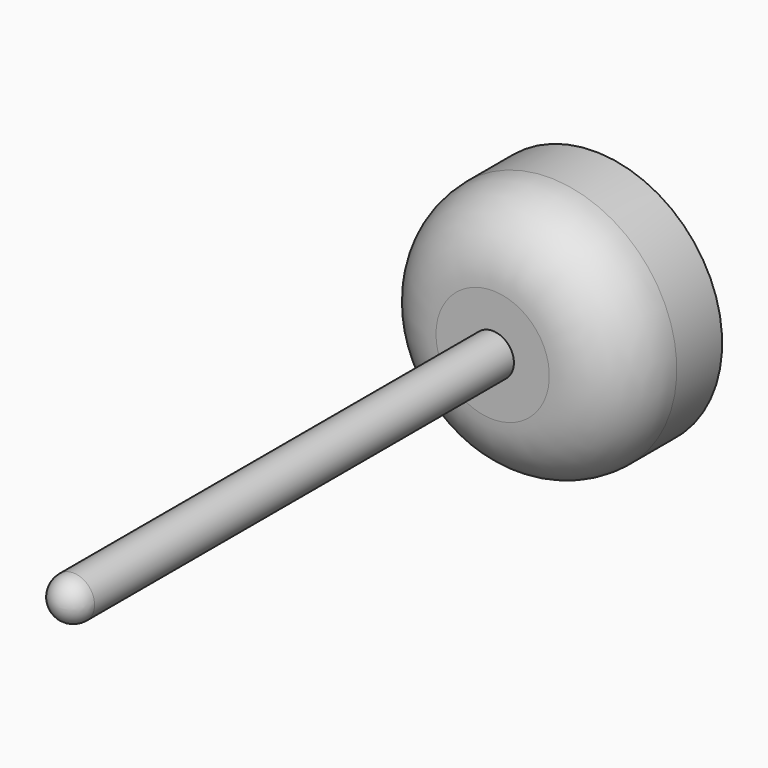
from build123d import *

# Parameters (mm, degrees)
F0_R     = 38.1
F1_DEPTH = 977.9
F2_R     = 38.1
F3_R     = 228.6
F4_DEPTH = 228.6
F5_T     = -25.4
F6_SIZE  = 50.8
F8_R     = 127
F9_SIZE  = 50.8
F10_R    = 76.2


# Not quite as in the source:
# - a fillet or chamfer that OpenCascade refuses, or shapes differently, is made with other operations: its cross-section is extruded or revolved along the edge and cut away or added


with BuildPart() as f1:
    # F0 (on Front) → F1 (new body)
    with BuildSketch(Plane.XZ):
        with Locations((-33.5694141686, 28.1756240875)):
            Circle(F0_R)
    extrude(amount=F1_DEPTH)

    # F2
    f2_edges = [f1.edges().sort_by_distance(p)[0] for p in [
        (-71.669414, -977.9, 28.175624),
    ]]
    fillet(f2_edges, radius=F2_R)


with BuildPart() as f4:
    # F3 (on face) → F4 (new body)
    with BuildSketch(Plane(origin=(0, 0, 0), x_dir=(-1, 0, 0), z_dir=(0, 1, 0))):
        with Locations((33.5694141686, 28.1756240875)):
            Circle(F3_R)
    extrude(amount=F4_DEPTH)

    # F5
    f5_openings = [f4.faces().sort_by_distance(p)[0] for p in [
        (-33.569414, 228.6, 28.175624),
    ]]
    offset(amount=F5_T, openings=f5_openings)

    # F6
    f6_edges = [f4.edges().sort_by_distance(p)[0] for p in [
        (169.630586, 25.4, 28.175624),
    ]]
    chamfer(f6_edges, length=F6_SIZE)

    # F7: chamfer of 50.8 on 3 edges, made by hand

    # F7_s1 → F7_t2 (revolve)
    with BuildSketch(Plane.XY.offset(28.1756240875)):
        Polygon((-221.8904386529, 61.3210244843), (-135.1694141686, 25.4), (-185.9694141686, 25.4), align=None)
    revolve(axis=Axis((-33.5694141686, 25.4, 28.1756240875), (0, -1, 0)))

    # F8
    f8_edges = [f4.edges().sort_by_distance(p)[0] for p in [
        (195.030586, 0, 28.175624),
    ]]
    fillet(f8_edges, radius=F8_R)

    # F9
    f9_edges = [f4.edges().sort_by_distance(p)[0] for p in [
        (68.030586, 25.4, 28.175624),
    ]]
    chamfer(f9_edges, length=F9_SIZE)

    # F10
    f10_edges = [f4.edges().sort_by_distance(p)[0] for p in [
        (-133.235954, 35.120159, 28.175624),
        (114.963666, 44.840318, 28.175624),
        (17.230586, 25.4, 28.175624),
    ]]
    fillet(f10_edges, radius=F10_R)


solid = Compound([f1.part, f4.part])
